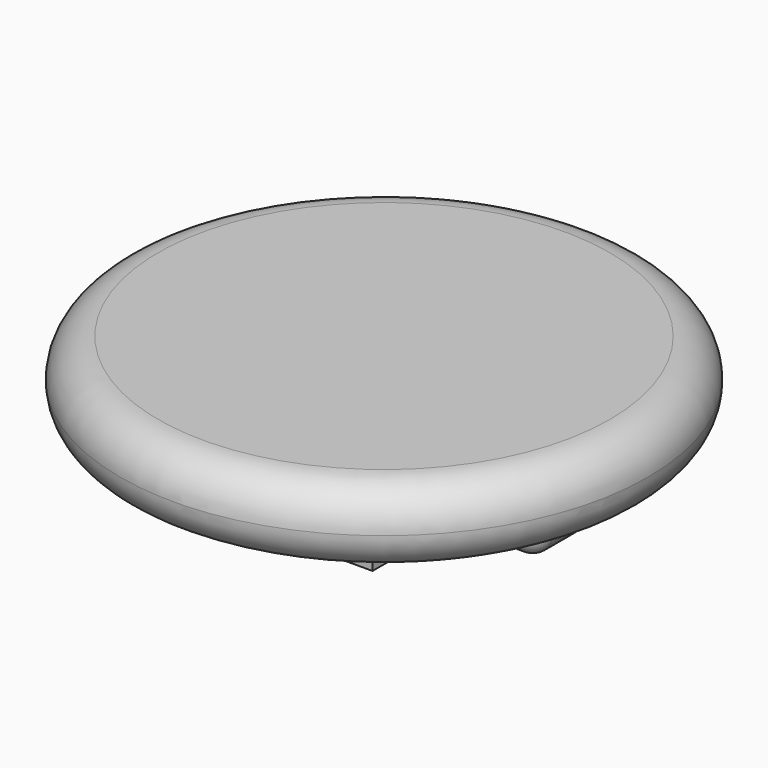
from build123d import *

# Parameters (mm, degrees)
F0_R     = 6.9
F1_DEPTH = 2
F2_R     = 0.99999
F3_W     = 5.4
F3_H     = 7.5
F4_DEPTH = 1
F5_W     = 7.9694418237
F5_H     = 1.9316775724
F6_DEPTH = 1
F7_R     = 0.5
F8_R     = 0.49999
F9_R     = 0.49999


# Not quite as in the source:
# - a fillet or chamfer is up to 0.001 mm smaller than in the source, because OpenCascade refuses the exact size


with BuildPart() as f1:
    # F0 (on Top) → F1 (new body)
    with BuildSketch(Plane.XY):
        Circle(F0_R)
    extrude(amount=F1_DEPTH)

    # F2 (radius 1 in the source; OpenCascade refuses exactly that, so slightly less here)
    f2_edges = [f1.edges().sort_by_distance(p)[0] for p in [
        (6.9, 0, 1),
        (-6.9, 0, 0),
        (-6.9, 0, 2),
    ]]
    fillet(f2_edges, radius=F2_R)

    # F3 (on face) → F4 (join)
    with BuildSketch(Plane.XY):
        Rectangle(F3_W, F3_H)
    extrude(amount=-F4_DEPTH)

    # F5 (on face) → F6 (join)
    with BuildSketch(Plane(origin=(0, 0, -1), x_dir=(1, 0, 0), z_dir=(0, 0, -1))):
        with Locations((0, -0.9658387862)):
            Rectangle(F5_W, F5_H)
    extrude(amount=F6_DEPTH)

    # F7
    f7_edges = [f1.edges().sort_by_distance(p)[0] for p in [
        (0, 0, -2),
        (0, 1.931678, -2),
    ]]
    fillet(f7_edges, radius=F7_R)

    # F8 (radius 0.5 in the source; OpenCascade refuses exactly that, so slightly less here)
    f8_edges = [f1.edges().sort_by_distance(p)[0] for p in [
        (-3.984721, 0.965839, -1),
        (-3.984721, 0.965839, -2),
    ]]
    fillet(f8_edges, radius=F8_R)

    # F9 (radius 0.5 in the source; OpenCascade refuses exactly that, so slightly less here)
    f9_edges = [f1.edges().sort_by_distance(p)[0] for p in [
        (3.984721, 0.965839, -2),
        (3.984721, 0.965839, -1),
    ]]
    fillet(f9_edges, radius=F9_R)


solid = f1.part
